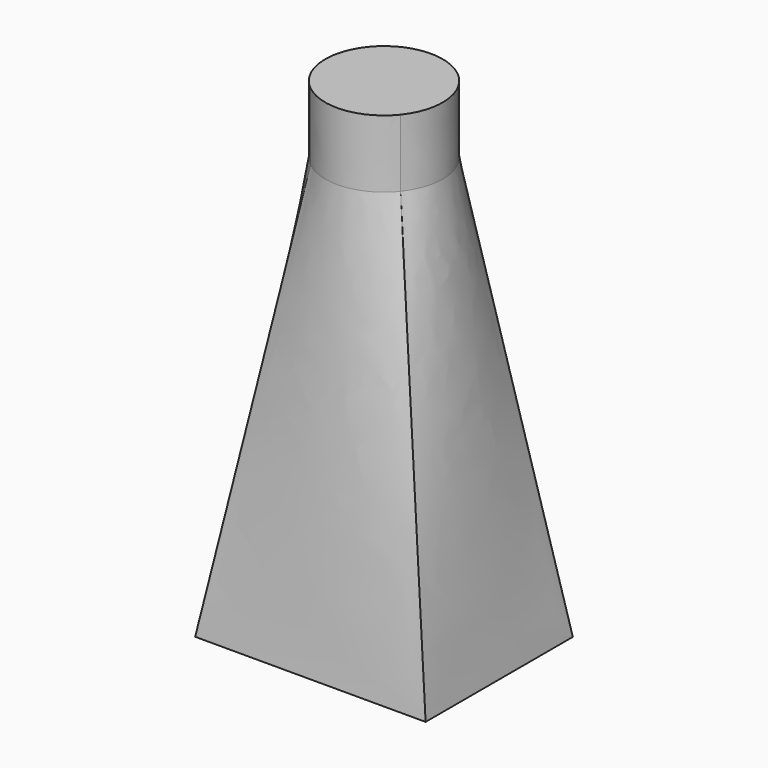
from build123d import *

# Parameters (mm, degrees)
F0_W     = 54.6039789915
F0_H     = 43.6073467135
F5_DEPTH = 16


# Not quite as in the source:
# - the arcs of a loft's sections are written as splines that run evenly, so that the points pair up as in the source's solid


with BuildPart() as f4:
    # F0 (on Top) → F4 section 0
    with BuildSketch(Plane.XY):
        Rectangle(F0_W, F0_H)
    # F3 (on offset) → F4 section 1
    with BuildSketch(Plane.XY.offset(100)):
        with BuildLine():
            add(Edge.make_bspline(
                [(10.8703523008, -8.681184603), (12.0067167081, -7.2582588142), (12.8597078303, -5.6099448874), (13.8703752153, -2.1109851988), (14.0276538234, -0.2617161283), (13.6223948312, 3.3576667769), (13.0600166829, 5.1263565389), (11.3005283214, 8.3151444232), (10.1041103917, 9.7339878936), (8.681184603, 10.8703523008)],
                knots=[0, 0, 0, 0, 0.25, 0.25, 0.5, 0.5, 0.75, 0.75, 1, 1, 1, 1], degree=3))
            add(Edge.make_bspline(
                [(8.681184603, 10.8703523008), (7.2582588142, 12.0067167081), (5.6099448874, 12.8597078303), (2.1109851988, 13.8703752153), (0.2617161283, 14.0276538234), (-3.3576667769, 13.6223948312), (-5.1263565389, 13.0600166829), (-8.3151444232, 11.3005283214), (-9.7339878936, 10.1041103917), (-10.8703523008, 8.681184603)],
                knots=[0, 0, 0, 0, 0.25, 0.25, 0.5, 0.5, 0.75, 0.75, 1, 1, 1, 1], degree=3))
            add(Edge.make_bspline(
                [(-10.8703523008, 8.681184603), (-12.0067167081, 7.2582588142), (-12.8597078303, 5.6099448874), (-13.8703752153, 2.1109851988), (-14.0276538234, 0.2617161283), (-13.6223948312, -3.3576667769), (-13.0600166829, -5.1263565389), (-11.3005283214, -8.3151444232), (-10.1041103917, -9.7339878936), (-8.681184603, -10.8703523008)],
                knots=[0, 0, 0, 0, 0.25, 0.25, 0.5, 0.5, 0.75, 0.75, 1, 1, 1, 1], degree=3))
            add(Edge.make_bspline(
                [(-8.681184603, -10.8703523008), (-7.2582588142, -12.0067167081), (-5.6099448874, -12.8597078303), (-2.1109851988, -13.8703752153), (-0.2617161283, -14.0276538234), (3.3576667769, -13.6223948312), (5.1263565389, -13.0600166829), (8.3151444232, -11.3005283214), (9.7339878936, -10.1041103917), (10.8703523008, -8.681184603)],
                knots=[0, 0, 0, 0, 0.25, 0.25, 0.5, 0.5, 0.75, 0.75, 1, 1, 1, 1], degree=3))
        make_face()
    loft(ruled=True)

    # F5 (add): a face of the model
    f5_faces = [f4.faces().sort_by_distance(p)[0] for p in [
        (0, 0, 100),
    ]]
    extrude(f5_faces, amount=F5_DEPTH)


solid = f4.part
